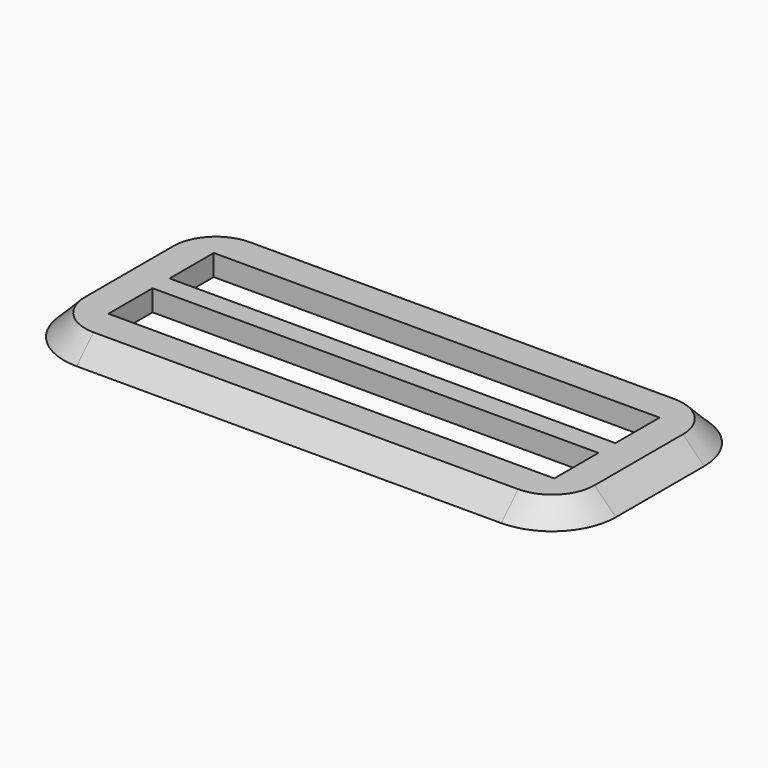
from build123d import *

# Parameters (mm, degrees)
F0_W     = 26
F0_H     = 11.2
F0_W_2   = 21
F0_H_2   = 2.6
F1_DEPTH = 1
F2_R     = 3
F3_SIZE  = 0.99999


# Not quite as in the source:
# - a fillet or chamfer is up to 0.001 mm smaller than in the source, because OpenCascade refuses the exact size


with BuildPart() as f1:
    # F0 (on Top) → F1 (new body)
    with BuildSketch(Plane.XY):
        Rectangle(F0_W, F0_H)
        with Locations((0, -1.8)):
            Rectangle(F0_W_2, F0_H_2, mode=Mode.SUBTRACT)
        with Locations((0, 1.8)):
            Rectangle(F0_W_2, F0_H_2, mode=Mode.SUBTRACT)
    extrude(amount=F1_DEPTH)

    # F2
    f2_edges = [f1.edges().sort_by_distance(p)[0] for p in [
        (-13, 5.6, 0.5),
        (-13, -5.6, 0.5),
        (13, -5.6, 0.5),
        (13, 5.6, 0.5),
    ]]
    fillet(f2_edges, radius=F2_R)

    # F3 (size 1 in the source; OpenCascade refuses exactly that, so slightly less here)
    f3_edges = [f1.edges().sort_by_distance(p)[0] for p in [
        (-12.12132, -4.72132, 1),
    ]]
    chamfer(f3_edges, length=F3_SIZE)


solid = f1.part
